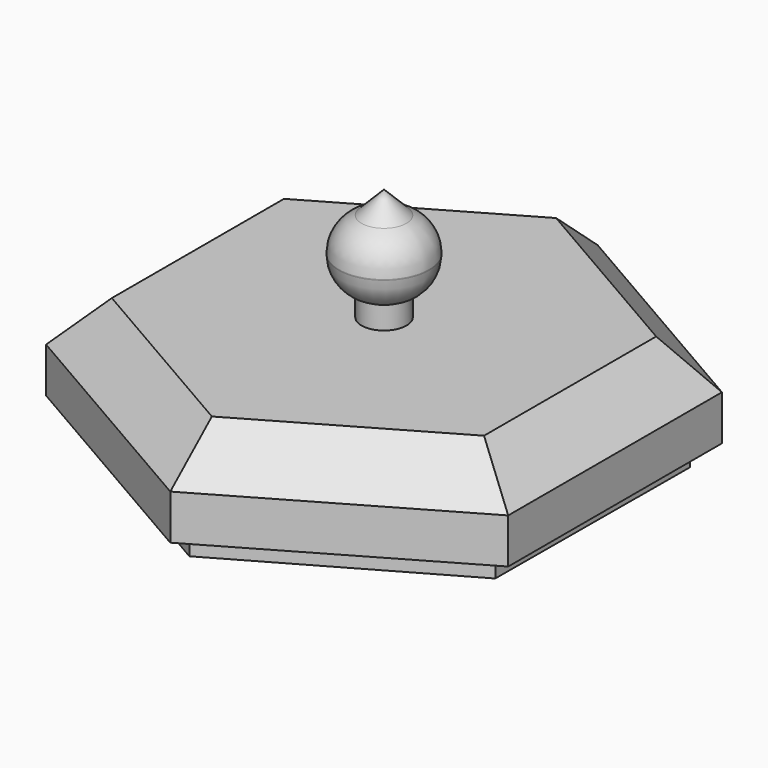
from build123d import *

# Parameters (mm, degrees)
F1_DEPTH  = 25.4
F2_SIZE   = 12.7
F3_R      = 6.35
F4_DEPTH  = 6.35
F5_R      = 12.7
F5_R_2    = 6.35
F6_DEPTH  = 19.05
F8_DEPTH  = 25.4
F9_SIZE   = 6.35
F11_DEPTH = 6.35
F12_T     = -2.54


# Not quite as in the source:
# - a fillet or chamfer that OpenCascade refuses, or shapes differently, is made with other operations: its cross-section is extruded or revolved along the edge and cut away or added


with BuildPart() as f1:
    # F0 (on Top) → F1 (new body)
    with BuildSketch(Plane.XY):
        Polygon((-0.0479153058, -75.3485536492), (65.2298039457, -37.7157726967), (65.2777192516, 37.6327809526), (0.0479153058, 75.3485536492), (-65.2298039457, 37.7157726967), (-65.2777192516, -37.6327809526), align=None)
    extrude(amount=F1_DEPTH)

    # F2
    f2_edges = [f1.edges().sort_by_distance(p)[0] for p in [
        (-32.662817, -56.490667, 25.4),
        (32.590944, -56.532163, 25.4),
        (65.253762, -0.041496, 25.4),
        (32.662817, 56.490667, 25.4),
        (-32.590944, 56.532163, 25.4),
        (-65.253762, 0.041496, 25.4),
    ]]
    chamfer(f2_edges, length=F2_SIZE)

    # F3 (on face) → F4 (join)
    with BuildSketch(Plane.XY.offset(25.4)):
        Circle(F3_R)
    extrude(amount=F4_DEPTH)


with BuildPart() as f6:
    # F5 (on face) → F6 (new body)
    with BuildSketch(Plane.XY.offset(31.75)):
        Circle(F5_R)
        Circle(F5_R_2, mode=Mode.SUBTRACT)
    extrude(amount=F6_DEPTH)

    # F7: fillet of radius 10.16 on 2 edges, made by hand

    # F7_s1 → F7_t2 (revolve, cut)
    with BuildSketch(Plane.XZ):
        with BuildLine():
            ThreePointArc((12.7, 41.3814279214), (10.9642269675, 47.0610405842), (6.35, 50.8))
            Line((6.35, 50.8), (12.7, 50.8))
            Line((12.7, 50.8), (12.7, 41.3814279214))
        make_face()
    revolve(axis=Axis((0, 0, 50.8), (0, 0, 1)), mode=Mode.SUBTRACT)

    # F7_s3 → F7_t4 (revolve, cut)
    with BuildSketch(Plane.XZ):
        with BuildLine():
            ThreePointArc((12.7, 41.1685720786), (10.9642269675, 35.4889594158), (6.35, 31.75))
            Line((6.35, 31.75), (12.7, 31.75))
            Line((12.7, 31.75), (12.7, 41.1685720786))
        make_face()
    revolve(axis=Axis((0, 0, 31.75), (0, 0, 1)), mode=Mode.SUBTRACT)


with BuildPart() as f8:
    # F8 (new): a face of the model
    f8_faces = [f1.part.faces().sort_by_distance(p)[0] for p in [
        (0, 0, 31.75),
    ]]
    extrude(f8_faces, amount=F8_DEPTH)

    # F9
    f9_edges = [f8.edges().sort_by_distance(p)[0] for p in [
        (-6.35, 0, 57.15),
    ]]
    chamfer(f9_edges, length=F9_SIZE)


with BuildPart() as f1_1:
    add(f1.part)

    # F10 (on face) → F11 (join)
    with BuildSketch(Plane(origin=(0, 0, 0), x_dir=(1, 0, 0), z_dir=(0, 0, -1))):
        Polygon((58.9554861724, 34.4266958261), (-0.3366500675, 68.2702966308), (-59.29213624, 33.8436008047), (-58.9554861724, -34.4266958261), (0.3366500675, -68.2702966308), (59.29213624, -33.8436008047), align=None)
    extrude(amount=F11_DEPTH)

    # F12
    f12_openings = [f1_1.faces().sort_by_distance(p)[0] for p in [
        (0, 0, -6.35),
    ]]
    offset(amount=F12_T, openings=f12_openings, kind=Kind.INTERSECTION)


solid = Compound([f6.part, f8.part, f1_1.part])
